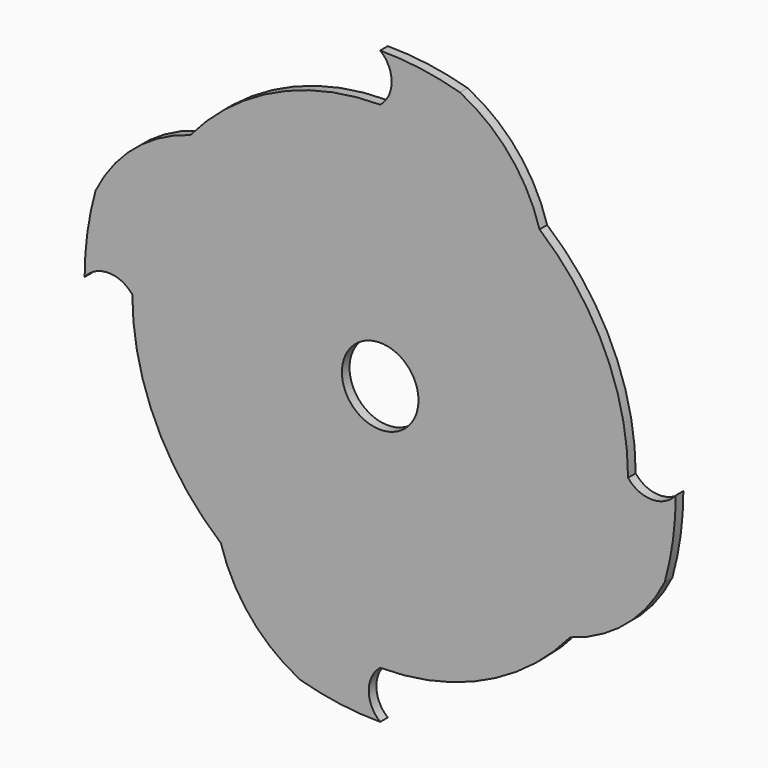
from build123d import *

# Parameters (mm, degrees)
F0_R            = 49.2125
F0_R_2          = 6.3754
F1_DEPTH        = 0.79375
F3_DEPTH        = 25.4
F3_DEPTH_BACK   = 25.4
F3_COPIES_COUNT = 4


# Not quite as in the source:
# - a pattern or mirror of a feature is missing from the dataset's text; its kind, count and spacing are read off the source's solid


with BuildPart() as f1:
    # F0 (on Front) → F1 (new body, symmetric)
    with BuildSketch(Plane.XZ):
        Circle(F0_R)
        Circle(F0_R_2, mode=Mode.SUBTRACT)
    extrude(amount=F1_DEPTH, both=True)

    # F2 (on Front) → F3 (cut, two sides)
    with BuildSketch(Plane.XZ) as f3_sk:
        with BuildLine():
            ThreePointArc((-31.6184843897, 26.5310585898), (-17.4435687533, 37.4078539099), (0, 41.275))
            ThreePointArc((0, 41.275), (1.9074798635, 45.24375), (0, 49.2125))
            ThreePointArc((0, 49.2125), (-29.7323648162, 39.2155152801), (-47.3851158452, 13.2861187933))
            ThreePointArc((-47.3851158452, 13.2861187933), (-40.9041876583, 21.5779754803), (-31.6184843897, 26.5310585898))
        make_face()
    f3 = extrude(amount=-F3_DEPTH, mode=Mode.SUBTRACT) + extrude(f3_sk.sketch, amount=F3_DEPTH_BACK, mode=Mode.SUBTRACT)

    # F3_copies: F3 ×4 about axis
    f3_copies_axis = Axis((0, 0, 0), (0, 1, 0))
    for i in range(1, F3_COPIES_COUNT):
        add(f3.rotate(f3_copies_axis, i * 360 / F3_COPIES_COUNT), mode=Mode.SUBTRACT)


solid = f1.part
